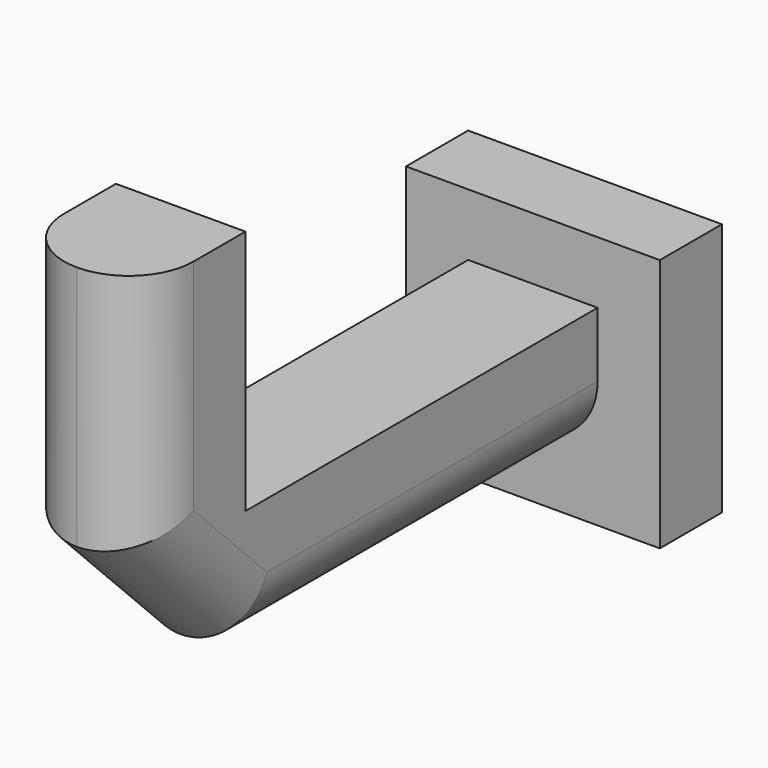
from build123d import *

# Parameters (mm, degrees)
F0_W     = 9.8
F0_H     = 9.8
F2_DEPTH = 3
F1_W     = 17
F1_H     = 5
F3_DEPTH = 2.5
F4_R     = 2.49999


# Not quite as in the source:
# - a fillet or chamfer is up to 0.001 mm smaller than in the source, because OpenCascade refuses the exact size


with BuildPart() as f2:
    # F0 (on Front) → F2 (new body)
    with BuildSketch(Plane.XZ):
        Rectangle(F0_W, F0_H)
    extrude(amount=-F2_DEPTH)

    # F1 (on Right) → F3 (join, symmetric)
    with BuildSketch(Plane.YZ):
        with Locations((-8.5, 0)):
            Rectangle(F1_W, F1_H)
        Polygon((-17, -2.5), (-17, 2.5), (-17, 12), (-22, 12), (-22, 2.5), align=None)
    extrude(amount=F3_DEPTH, both=True)

    # F4 (radius 2.5 in the source; OpenCascade refuses exactly that, so slightly less here)
    f4_edges = [f2.edges().sort_by_distance(p)[0] for p in [
        (-2.5, -8.5, -2.5),
        (-2.5, -19.5, 0),
        (2.5, -8.5, -2.5),
        (2.5, -19.5, 0),
        (2.5, -22, 7.25),
        (-2.5, -22, 7.25),
    ]]
    fillet(f4_edges, radius=F4_R)


solid = f2.part
